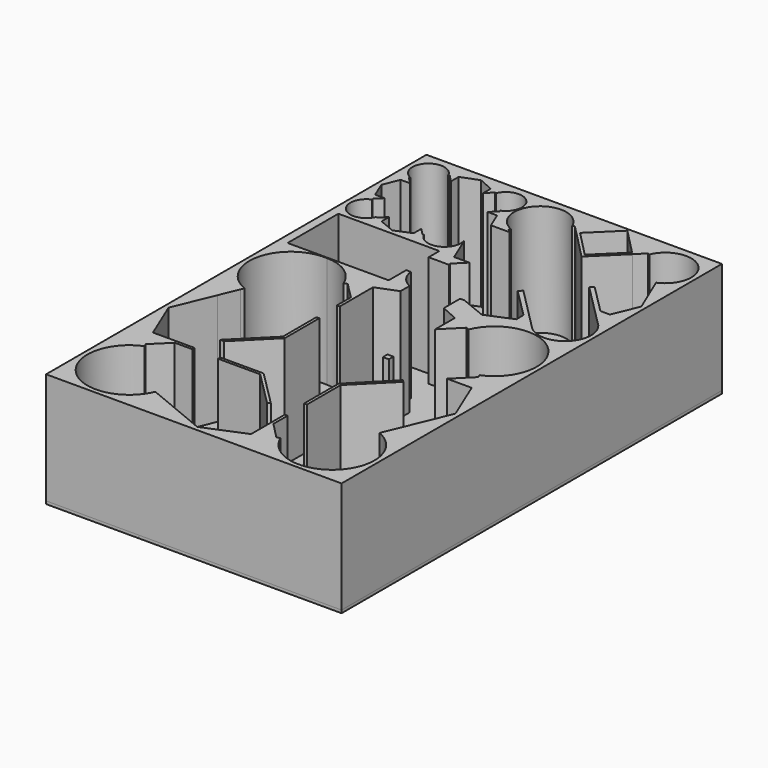
from build123d import *

# Parameters (mm, degrees)
F0_W     = 10341.299638
F0_H     = 16639.522815
F1_DEPTH = 4000
F0_W_2   = 208.580964
F0_H_2   = 199.637335
F2_W     = 16639.522815
F2_H     = 100
F3_DEPTH = 10341.299638


# Not quite as in the source:
# - ends of sketch curves that miss each other by under 0.0002 mm in the source are joined


with BuildPart() as f1:
    # F0 (on Top) → F1 (new body)
    with BuildSketch(Plane.XY):
        with Locations((0, 5e-07)):
            Rectangle(F0_W, F0_H)
        with BuildLine():
            Line((1903.589092, 6260.567045), (2904.542439, 7239.388988))
            Line((2904.542439, 7239.388988), (3203.094187, 7544.712283))
            Line((3203.094187, 7544.712283), (3272.270672, 7516.058423))
            ThreePointArc((3272.270672, 7516.058423), (4754.4756925814, 7810.8882666211), (4459.6463241165, 6328.6831517187))
            Line((4459.6463241165, 6328.6831517187), (4488.300572, 6259.505676))
            Line((4488.300572, 6259.505676), (4644.221467, 5883.079336))
            Line((4644.221467, 5883.079336), (5029.540868, 4974.29626))
            Line((5029.540868, 4974.29626), (4653.113113, 4065.523015))
            Line((4653.113113, 4065.523015), (4644.222437, 4065.5230015785))
            Line((4644.222437, 4065.5230015785), (4321.240219, 4065.522514))
            Line((4321.240219, 4065.522514), (3309.305349, 5080.222097))
            Line((3309.305349, 5080.222097), (3203.206295, 4974.186433))
            Line((3203.206295, 4974.186433), (4808.375986, 3364.633825))
            ThreePointArc((4808.375986, 3364.633825), (4753.5332453491, 2136.4626260677), (3525.3620232337, 2081.6204152797))
            Line((3525.3620232337, 2081.6204152797), (1922.334351, 3693.539458))
            Line((1922.334351, 3693.539458), (1811.823039, 3583.028057))
            Line((1811.823039, 3583.028057), (2826.666463, 2568.184196))
            Line((2826.666463, 2568.184196), (2835.557139, 2251.649196))
            Line((2835.557139, 2251.649196), (1926.779323, 1871.538461))
            Line((1926.779323, 1871.538461), (1009.111173, 2247.966415))
            Line((1009.111173, 2247.966415), (870.537575, 2239.349513))
            Line((870.537575, 2239.349513), (870.537575, 1529.148136))
            Line((870.537575, 1529.148136), (1470.514286, 1262.431955))
            Line((1470.514286, 1262.431955), (1470.514286, 401.025281))
            Line((1470.514286, 401.025281), (2079.620645, 1010.13164))
            Line((2079.620645, 1010.13164), (2189.276828, 964.710526))
            ThreePointArc((2189.276828, 964.710526), (4591.692983169, 1442.5794731284), (4113.8223201326, -959.8363413202))
            Line((4113.8223201326, -959.8363413202), (4159.242656, -1069.490732))
            Line((4159.242656, -1069.490732), (3550.138249, -1678.595139))
            Line((3550.138249, -1678.595139), (4411.541962, -1678.595139))
            Line((4411.541962, -1678.595139), (5020.649819, -3149.117648))
            Line((5020.649819, -3149.117648), (4411.543411, -4619.624538))
            Line((4411.543411, -4619.624538), (4159.242854, -5228.731964))
            Line((4159.242854, -5228.731964), (4113.822405, -5338.38713))
            ThreePointArc((4113.822405, -5338.38713), (4591.6927084572, -7740.8031838403), (2189.2765651834, -7262.9333293382))
            Line((2189.2765651834, -7262.9333293382), (2079.621061, -7308.354158))
            Line((2079.621061, -7308.354158), (1514.76035, -6730.919773))
            Line((1514.76035, -6730.919773), (1514.76035, -6110.919773))
            Line((1514.76035, -6110.919773), (1414.76035, -6110.919773))
            Line((1414.76035, -6110.919773), (1414.76035, -7583.748482))
            Line((1414.76035, -7583.748482), (0, -8169.761407))
            Line((0, -8169.761407), (-1470.513733, -7560.654675))
            Line((-1470.513733, -7560.654675), (-2079.620855, -7308.354243))
            Line((-2079.620855, -7308.354243), (-2191.557204, -7261.98864))
            ThreePointArc((-2191.557204, -7261.98864), (-4589.946951546, -7739.0574546245), (-4112.8778162627, -5340.6677713657))
            Line((-4112.8778162627, -5340.6677713657), (-4159.243115, -5228.732119))
            Line((-4159.243115, -5228.732119), (-3591.244857, -4665.941899))
            Line((-3591.244857, -4665.941899), (-2971.244857, -4665.941899))
            Line((-2971.244857, -4665.941899), (-2971.244857, -4565.941899))
            Line((-2971.244857, -4565.941899), (-4433.779923, -4565.941899))
            Line((-4433.779923, -4565.941899), (-5020.649612, -3149.111588))
            Line((-5020.649612, -3149.111588), (-4434.25464, -1733.429529))
            Line((-4434.25464, -1733.429529), (-4159.241373, -1069.489068))
            Line((-4159.241373, -1069.489068), (-4159.241555, -1069.488855))
            Line((-4159.241555, -1069.488855), (-4113.820899, -959.833634))
            ThreePointArc((-4113.820899, -959.833634), (-4987.7485519057, 718.4797689086), (-3464.8484919602, 1841.5384615497))
            ThreePointArc((-3464.8484919602, 1841.5384615497), (-2692.5827745251, 1598.7596156767), (-2189.2748820581, 964.7114539772))
            Line((-2189.2748820581, 964.7114539772), (-2079.618819, 1010.132397))
            Line((-2079.618819, 1010.132397), (-1511.625946, 442.13928))
            Line((-1511.625946, 442.13928), (-1511.625558, -165.805426))
            Line((-1511.625558, -165.805426), (-1411.625558, -165.805426))
            Line((-1411.625558, -165.805426), (-1411.62616, 1285.266228))
            Line((-1411.62616, 1285.266228), (-680.218687, 1568.874278))
            Line((-680.218687, 1568.874278), (-680.218687, 1871.538461))
            Line((-680.218687, 1871.538461), (-680.218687, 1966.337642))
            ThreePointArc((-680.218687, 1966.337642), (-1014.8790423033, 2238.6659951889), (-1173.9350191528, 2639.7414019812))
            Line((-1173.9350191528, 2639.7414019812), (-1334.872756, 2639.741402))
            Line((-1334.872756, 2639.741402), (-1334.872756, 1871.538461))
            Line((-1334.872756, 1871.538461), (-4870.64959, 1871.538461))
            Line((-4870.64959, 1871.538461), (-4870.64959, 4091.284946))
            Line((-4870.64959, 4091.284946), (-1334.872756, 4091.284946))
            Line((-1334.872756, 4091.284946), (-1334.872756, 3619.918202))
            Line((-1334.872756, 3619.918202), (-1184.872756, 3619.918202))
            Line((-1184.872756, 3619.918202), (-623.869765, 3619.918202))
            Line((-623.869765, 3619.918202), (-643.632885, 3689.094535))
            Line((-643.632885, 3689.094535), (-267.204405, 4065.523015))
            Line((-267.204405, 4065.523015), (-799.55475, 4065.523015))
            Line((-799.55475, 4065.523015), (-1175.981054, 4974.300005))
            Line((-1175.981054, 4974.300005), (-1184.87173, 4974.300005))
            ThreePointArc((-1184.87173, 4974.300005), (-1544.9588604922, 4276.7815166727), (-2265.5864419615, 4588.0541810168))
            Line((-2265.5864419615, 4588.0541810168), (-2308.346139, 4570.342522))
            Line((-2308.346139, 4570.342522), (-2541.024933, 4803.021416))
            Line((-2541.024933, 4803.021416), (-2541.024933, 4473.96381))
            Line((-2541.024933, 4473.96381), (-3102.761403, 4241.284946))
            Line((-3102.761403, 4241.284946), (-3664.497662, 4473.963723))
            Line((-3664.497662, 4473.963723), (-3664.497662, 4803.021416))
            Line((-3664.497662, 4803.021416), (-3897.176588, 4570.34249))
            Line((-3897.176588, 4570.34249), (-3939.936336, 4588.054177))
            ThreePointArc((-3939.936336, 4588.054177), (-4856.1211301684, 4405.8139061021), (-4673.8807388704, 5321.9986766871))
            Line((-4673.8807388704, 5321.9986766871), (-4691.592309, 5364.758159))
            Line((-4691.592309, 5364.758159), (-4458.913207, 5597.437261))
            Line((-4458.913207, 5597.437261), (-4787.9712, 5597.437261))
            Line((-4787.9712, 5597.437261), (-5020.648956, 6159.173221))
            Line((-5020.648956, 6159.173221), (-4796.646714, 6720.910517))
            Line((-4796.646714, 6720.910517), (-4458.913207, 6720.910517))
            Line((-4458.913207, 6720.910517), (-4691.591713, 6953.589123))
            Line((-4691.591713, 6953.589123), (-4674.044624, 6995.951566))
            ThreePointArc((-4674.044624, 6995.951566), (-4851.2840085015, 7907.2438267655), (-3939.9357195462, 7730.2927571927))
            Line((-3939.9357195462, 7730.2927571927), (-3897.17581, 7748.004459))
            Line((-3897.17581, 7748.004459), (-3664.496476, 7515.325025))
            Line((-3664.496476, 7515.325025), (-3664.497662, 7844.38298))
            Line((-3664.497662, 7844.38298), (-3064.434282, 8077.061495))
            Line((-3064.434282, 8077.061495), (-2541.024933, 7844.382892))
            Line((-2541.024933, 7844.382892), (-2541.024933, 7515.325535))
            Line((-2541.024933, 7515.325535), (-2308.346298, 7748.00417))
            Line((-2308.346298, 7748.00417), (-2265.586568, 7730.292495))
            ThreePointArc((-2265.586568, 7730.292495), (-1349.4017201593, 7912.5327912257), (-1531.6422740976, 6996.3479952357))
            Line((-1531.6422740976, 6996.3479952357), (-1513.930672, 6953.588406))
            Line((-1513.930672, 6953.588406), (-1746.608561, 6720.910517))
            Line((-1746.608561, 6720.910517), (-1417.552335, 6720.910517))
            Line((-1417.552335, 6720.910517), (-1184.873128, 6159.170906))
            Line((-1184.873128, 6159.170906), (-543.296034, 6159.170906))
            Line((-543.296034, 6159.170906), (-643.631921, 6259.506836))
            Line((-643.631921, 6259.506836), (-614.977499, 6328.684767))
            ThreePointArc((-614.977499, 6328.684767), (-915.1086587372, 7816.1900295466), (572.3964591582, 7516.0581520645))
            Line((572.3964591582, 7516.0581520645), (641.574912, 7544.712751))
            Line((641.574912, 7544.712751), (924.767149, 7261.520392))
            Line((924.767149, 7261.520392), (1903.589092, 6260.567045))
        make_face(mode=Mode.SUBTRACT)
        Polygon((996.263816, 7331.436245), (1925.720496, 8240.342335), (2834.626586, 7310.885656), (1905.169907, 6401.979565), align=None, mode=Mode.SUBTRACT)
    extrude(amount=F1_DEPTH)


with BuildPart() as f1b:
    # F0 (on Top) → F1, piece 2 (new body)
    with BuildSketch(Plane.XY):
        Polygon((2733.123826, -2571.524935), (2662.410198, -2500.811501), (2528.1429422139, -2635.0797392139), (1421.069783, -3755.833305), (1414.76035, -4189.5244096315), (1414.76035, -5260.470478), (1514.76035, -5260.470478), (1514.76035, -3789.891754), align=None)
    extrude(amount=F1_DEPTH)


with BuildPart() as f1c:
    # F0 (on Top) → F1, piece 3 (new body)
    with BuildSketch(Plane.XY):
        Polygon((-600.216725, -4665.941899), (618.149088, -5884.308237), (689.888544, -5814.626337), (54.6019528578, -5179.3394721422), (-558.795356, -4565.941899), (-1461.622004, -4565.942379), (-1461.6220040007, -4565.941899), (-2071.244857, -4565.941899), (-2071.244857, -4665.941899), align=None)
    extrude(amount=F1_DEPTH)


with BuildPart() as f1d:
    # F0 (on Top) → F1, piece 4 (new body)
    with BuildSketch(Plane.XY):
        Polygon((-2729.838154, -3754.535196), (-2588.416798, -3754.535196), (-2038.326382, -3204.44478), (-2025.019791, -3191.138189), (-1411.623013, -2577.741411), (-1411.6246032683, -1070.29071), (-1411.624608, -1065.805426), (-1511.624608, -1065.805426), (-1511.623057, -2536.320099), (-2110.707123, -3135.404165), align=None)
    extrude(amount=F1_DEPTH)


with BuildPart() as f1e:
    # F0 (on Top) → F1, piece 5 (new body)
    with BuildSketch(Plane.XY):
        with Locations((1484.891403, -1674.5140205)):
            Rectangle(F0_W_2, F0_H_2)
    extrude(amount=F1_DEPTH)


with BuildPart() as f3:
    # F2 (on face) → F3 (new body, through all)
    with BuildSketch(Plane.YZ.offset(5170.649819)):
        with Locations((5e-07, 50)):
            Rectangle(F2_W, F2_H)
    extrude(amount=-F3_DEPTH)


solid = Compound([f1.part, f1b.part, f1c.part, f1d.part, f1e.part, f3.part])
